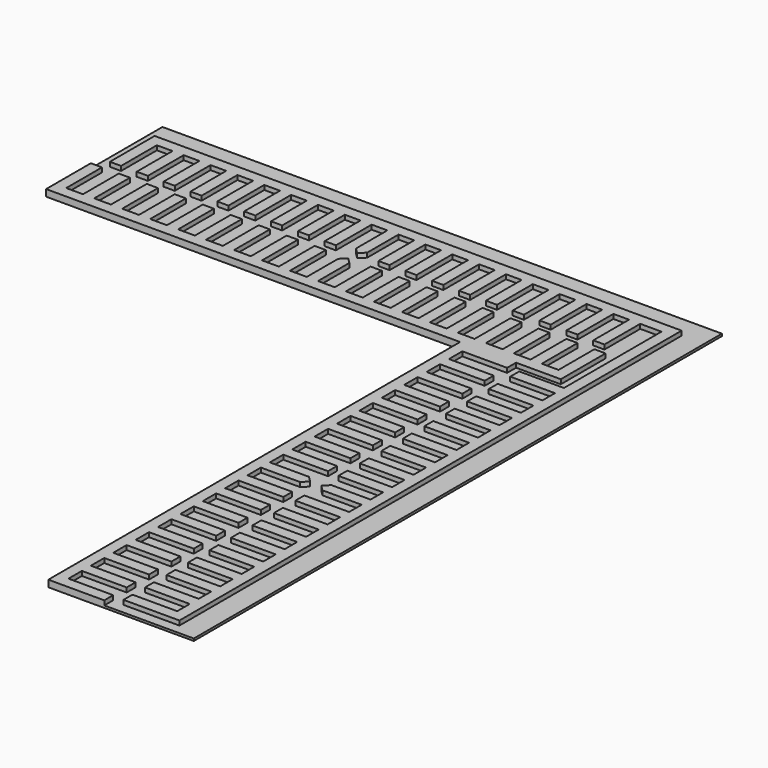
from build123d import *

# Parameters (mm, degrees)
F1_W      = 1
F1_H      = 4
F2_DEPTH  = 0.4
F3_W      = 1
F3_H      = 4
F4_DEPTH  = 0.4
F7_SIZE   = 0.49999
F7_2_SIZE = 0.49999
F8_ANGLE  = 90
F9_ANGLE  = 90
F12_DEPTH = 0.4
F14_DEPTH = 0.2


# Not quite as in the source:
# - a fillet or chamfer is up to 0.001 mm smaller than in the source, because OpenCascade refuses the exact size


with BuildPart() as f2:
    # F1 (on Top) → F2 (new body)
    with BuildSketch(Plane.XY):
        with Locations((0, 2)):
            Rectangle(F1_W, F1_H)
        Polygon((0.5, 0), (-0.5, 0), (-2, 0), (-3, 0), (-4.5, 0), (-5.5, 0), (-7, 0), (-8, 0), (-9.5, 0), (-10.5, 0), (-12, 0), (-13, 0), (-14.5, 0), (-15.5, 0), (-17, 0), (-18, 0), (-19.5, 0), (-20.5, 0), (-22, 0), (-23, 0), (-23, -1), (23, -1), (23, 0), (22, 0), (20.5, 0), (19.5, 0), (18, 0), (17, 0), (15.5, 0), (14.5, 0), (13, 0), (12, 0), (10.5, 0), (9.5, 0), (8, 0), (7, 0), (5.5, 0), (4.5, 0), (3, 0), (2, 0), align=None)
        with Locations((-2.5, 2)):
            Rectangle(F1_W, F1_H)
        with Locations((2.5, 2)):
            Rectangle(F1_W, F1_H)
        with Locations((-5, 2)):
            Rectangle(F1_W, F1_H)
        with Locations((5, 2)):
            Rectangle(F1_W, F1_H)
        with Locations((-7.5, 2)):
            Rectangle(F1_W, F1_H)
        with Locations((7.5, 2)):
            Rectangle(F1_W, F1_H)
        with Locations((-10, 2)):
            Rectangle(F1_W, F1_H)
        with Locations((10, 2)):
            Rectangle(F1_W, F1_H)
        with Locations((-12.5, 2)):
            Rectangle(F1_W, F1_H)
        with Locations((12.5, 2)):
            Rectangle(F1_W, F1_H)
        with Locations((-15, 2)):
            Rectangle(F1_W, F1_H)
        with Locations((15, 2)):
            Rectangle(F1_W, F1_H)
        with Locations((-17.5, 2)):
            Rectangle(F1_W, F1_H)
        with Locations((17.5, 2)):
            Rectangle(F1_W, F1_H)
        with Locations((-20, 2)):
            Rectangle(F1_W, F1_H)
        with Locations((20, 2)):
            Rectangle(F1_W, F1_H)
        with Locations((-22.5, 2)):
            Rectangle(F1_W, F1_H)
        with Locations((22.5, 2)):
            Rectangle(F1_W, F1_H)
    extrude(amount=F2_DEPTH)

    # F7 (size 0.5 in the source; OpenCascade refuses exactly that, so slightly less here)
    f7_edges = [f2.edges().sort_by_distance(p)[0] for p in [
        (0.5, 4, 0.2),
        (-0.5, 4, 0.2),
    ]]
    chamfer(f7_edges, length=F7_SIZE)


with BuildPart() as f4:
    # F3 (on Top) → F4 (new body)
    with BuildSketch(Plane.XY):
        with Locations((0, -7)):
            Rectangle(F3_W, F3_H)
        Polygon((0.5, -9), (-0.5, -9), (-1.9, -9), (-2.9, -9), (-4.3, -9), (-5.3, -9), (-6.7, -9), (-7.7, -9), (-9.1, -9), (-10.1, -9), (-11.5, -9), (-12.5, -9), (-13.9, -9), (-14.9, -9), (-16.3, -9), (-17.3, -9), (-18.7, -9), (-19.7, -9), (-21.1, -9), (-22.1, -9), (-22.1, -10), (22.1, -10), (22.1, -9), (21.1, -9), (19.7, -9), (18.7, -9), (17.3, -9), (16.3, -9), (14.9, -9), (13.9, -9), (12.5, -9), (11.5, -9), (10.1, -9), (9.1, -9), (7.7, -9), (6.7, -9), (5.3, -9), (4.3, -9), (2.9, -9), (1.9, -9), align=None)
        with Locations((-2.4, -7)):
            Rectangle(F3_W, F3_H)
        with Locations((2.4, -7)):
            Rectangle(F3_W, F3_H)
        with Locations((-4.8, -7)):
            Rectangle(F3_W, F3_H)
        with Locations((4.8, -7)):
            Rectangle(F3_W, F3_H)
        with Locations((-7.2, -7)):
            Rectangle(F3_W, F3_H)
        with Locations((7.2, -7)):
            Rectangle(F3_W, F3_H)
        with Locations((-9.6, -7)):
            Rectangle(F3_W, F3_H)
        with Locations((9.6, -7)):
            Rectangle(F3_W, F3_H)
        with Locations((-12, -7)):
            Rectangle(F3_W, F3_H)
        with Locations((12, -7)):
            Rectangle(F3_W, F3_H)
        with Locations((-14.4, -7)):
            Rectangle(F3_W, F3_H)
        with Locations((14.4, -7)):
            Rectangle(F3_W, F3_H)
        with Locations((-16.8, -7)):
            Rectangle(F3_W, F3_H)
        with Locations((16.8, -7)):
            Rectangle(F3_W, F3_H)
        with Locations((-19.2, -7)):
            Rectangle(F3_W, F3_H)
        with Locations((19.2, -7)):
            Rectangle(F3_W, F3_H)
        with Locations((-21.6, -7)):
            Rectangle(F3_W, F3_H)
        with Locations((21.6, -7)):
            Rectangle(F3_W, F3_H)
    extrude(amount=F4_DEPTH)


with BuildPart() as f5_1:
    # F5: instance of F4
    add(f4.part.mirror(Plane.XZ))

    # F7#2 (size 0.5 in the source; OpenCascade refuses exactly that, so slightly less here)
    f7_2_edges = [f5_1.edges().sort_by_distance(p)[0] for p in [
        (-0.5, 5, 0.2),
        (0.5, 5, 0.2),
    ]]
    chamfer(f7_2_edges, length=F7_2_SIZE)


with BuildPart() as f8_1:
    # F8: copy of F2
    add(f2.part.rotate(Axis((-23, -1, 0.2), (0, 0, -1)), F8_ANGLE))


with BuildPart() as f9_1:
    # F9: copy of F5_1
    add(f5_1.part.rotate(Axis((-23, -1, 0.2), (0, 0, -1)), F9_ANGLE))


with BuildPart() as f8_1_1:
    # F10: moved
    add(f8_1.part.moved(Location((37, 0, 0))))


with BuildPart() as f9_1_1:
    # F10: moved
    add(f9_1.part.moved(Location((37, 0, 0))))


with BuildPart() as f5_1_1:
    add(f5_1.part)

    add(f9_1_1.part)  # F12 merges F9_1
    # F11 (on Top) → F12 (join)
    with BuildSketch(Plane.XY):
        Polygon((24, -1.9), (25, -1.9), (25, 10), (22.1, 10), (22.1, 9), (24, 9), align=None)
    extrude(amount=F12_DEPTH)


with BuildPart() as f2_1:
    add(f2.part)

    add(f8_1_1.part)  # F14 merges F8_1
    # F13 (on Top) → F14 (join)
    with BuildSketch(Plane.XY):
        Polygon((-23, 12), (-23, -1), (14, -1), (14, -47), (27, -47), (27, 12), align=None)
    extrude(amount=-F14_DEPTH)


solid = Compound([f5_1_1.part, f2_1.part])
